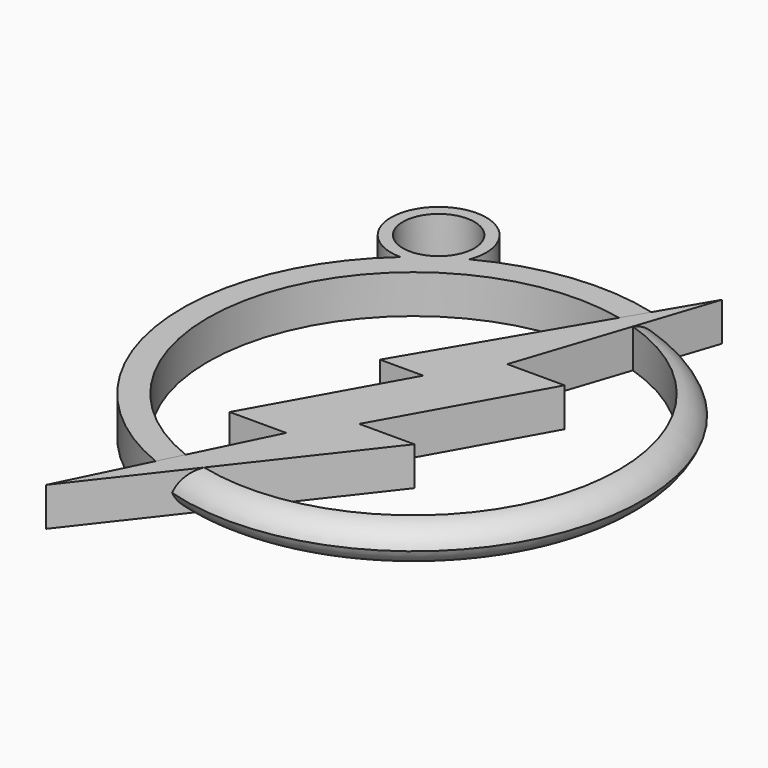
from build123d import *

# Parameters (mm, degrees)
F1_DEPTH    = 6.35
F3_DEPTH    = 6.35
F4_R        = 7.8194869238
F4_R_2      = 5.8680689484
F5_DEPTH    = 6.35
F6_T2_ANGLE = 216.8401406518
F6_T4_ANGLE = 216.8401406518


# Not quite as in the source:
# - a fillet or chamfer that OpenCascade refuses, or shapes differently, is made with other operations: its cross-section is extruded or revolved along the edge and cut away or added


with BuildPart() as f1:
    # F0 (on Top) → F1 (new body)
    with BuildSketch(Plane.XY):
        Polygon((10.2044390514, 20.2409497), (20.5251984298, 51.3899475336), (-3.3272264991, 11.0243037343), (3.7826313637, 11.0243037343), (-9.2903310433, -12.3694203794), (0, -12.3694203794), (-15.0240883231, -42.8730025887), (14.7914448753, -4.5715132728), (5.745598625, -4.5715132728), (19.6113856238, 20.2409497), align=None)
    extrude(amount=F1_DEPTH)


with BuildPart() as f3:
    # F2 (on face) → F3 (new body)
    with BuildSketch(Plane.XY.offset(6.35)):
        with BuildLine():
            ThreePointArc((-6.2910568685, -25.142226705), (-26.3355362631, 16.1610780131), (13.3489113778, 39.2454612683))
            Line((13.3489113778, 39.2454612683), (15.6022474373, 43.0587993675))
            ThreePointArc((15.6022474373, 43.0587993675), (-30.1282761074, 18.2224985015), (-8.1703070611, -28.9576903466))
            Line((-8.1703070611, -28.9576903466), (-6.2910568685, -25.142226705))
        make_face()
    extrude(amount=-F3_DEPTH)

    # F4 (on face) → F5 (join)
    with BuildSketch(Plane.XY.offset(6.35)):
        with Locations((-19.0615635365, 42.7367538214)):
            Circle(F4_R)
        with Locations((-19.0615635365, 42.7367538214)):
            Circle(F4_R_2, mode=Mode.SUBTRACT)
    extrude(amount=-F5_DEPTH)


with BuildPart() as f3b:
    # F2 (on face) → F3, piece 2 (new body)
    with BuildSketch(Plane.XY.offset(6.35)):
        with BuildLine():
            ThreePointArc((16.2408188754, 38.4592973202), (33.2131829481, 26.2118953895), (39.7023464178, 6.3133840449))
            ThreePointArc((39.7023464178, 6.3133840449), (26.7251834492, -20.2880192706), (-2.2275902486, -26.4344257227))
            Line((-2.2275902486, -26.4344257227), (-5.0447458233, -30.0533868002))
            ThreePointArc((-5.0447458233, -30.0533868002), (28.5956235275, -24.1914535774), (43.9413588571, 6.3133840449))
            ThreePointArc((43.9413588571, 6.3133840449), (36.6498565452, 28.693610287), (17.57413441, 42.4833658191))
            Line((17.57413441, 42.4833658191), (16.2408188754, 38.4592973202))
        make_face()
    extrude(amount=-F3_DEPTH)

    # F6: fillet of radius 5.08 on 2 edges, made by hand

    # F6_s1 → F6_t2 (revolve, cut)
    with BuildSketch(Plane(origin=(6.0682659835, 0.1166447559, 0), x_dir=(0, 0, 1), z_dir=(-0.9998153068, -0.01921854, 0))):
        with BuildLine():
            ThreePointArc((6.35, 39.9510787116), (4.6214204879, 42.98814587), (1.340095817, 44.190091151))
            Line((1.340095817, 44.190091151), (6.35, 44.190091151))
            Line((6.35, 44.190091151), (6.35, 39.9510787116))
        make_face()
    revolve(axis=Axis((5.9491517022, 6.3133840449, 6.35), (0, 0, -1)), revolution_arc=F6_T2_ANGLE, mode=Mode.SUBTRACT)

    # F6_s3 → F6_t4 (revolve, cut)
    with BuildSketch(Plane(origin=(0.9263339106, -0.6665933412, 0), x_dir=(0, 0, 1), z_dir=(-0.8116868319, 0.5840928752, 0))):
        with BuildLine():
            ThreePointArc((0, -25.1538468985), (1.7285795121, -28.1909140569), (5.009904183, -29.3928593379))
            Line((5.009904183, -29.3928593379), (0, -29.3928593379))
            Line((0, -29.3928593379), (0, -25.1538468985))
        make_face()
    revolve(axis=Axis((5.9491517022, 6.3133840449, 0), (0, 0, 1)), revolution_arc=F6_T4_ANGLE, mode=Mode.SUBTRACT)


solid = Compound([f1.part, f3.part, f3b.part])
